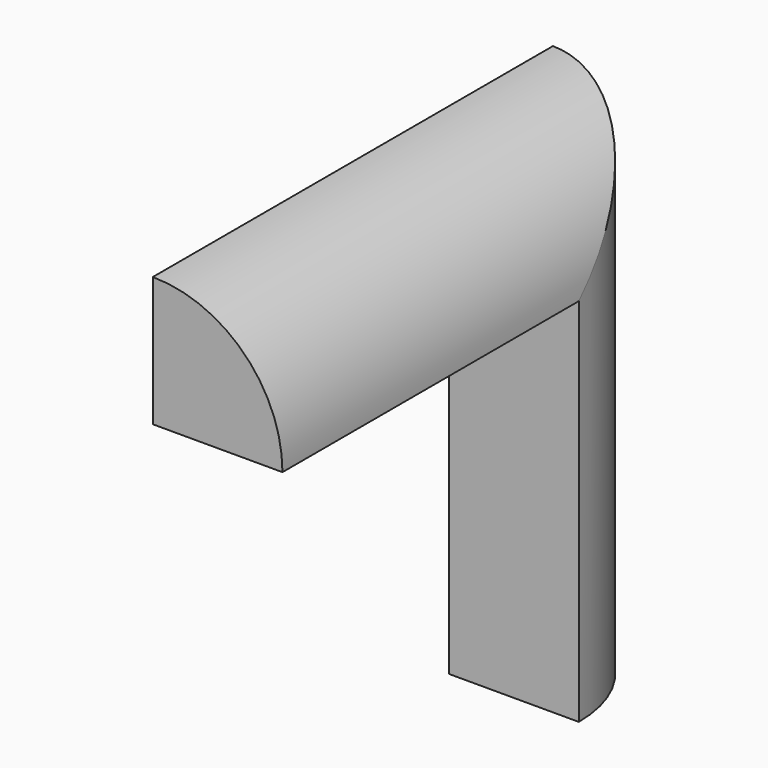
from build123d import *

# Parameters (mm, degrees)
F1_DEPTH      = 15
F3_DEPTH      = 15
F3_DEPTH_BACK = 7
F6_DEPTH      = 20
F7_DEPTH      = 20


with BuildPart() as f1:
    # F0 (on Top) → F1 (new body)
    with BuildSketch(Plane.XY):
        with BuildLine():
            Line((0, 0), (7, 0))
            ThreePointArc((7, 0), (4.9497474683, 4.9497474683), (0, 7))
            Line((0, 7), (0, 0))
        make_face()
    extrude(amount=F1_DEPTH)


with BuildPart() as f3:
    # F2 (on face) → F3 (new body, two sides)
    with BuildSketch(Plane.XZ) as f3_sk:
        with BuildLine():
            ThreePointArc((7, 8), (4.9497474683, 12.9497474683), (0, 15))
            Line((0, 15), (0, 8))
            Line((0, 8), (7, 8))
        make_face()
    extrude(amount=F3_DEPTH)
    extrude(f3_sk.sketch, amount=-F3_DEPTH_BACK)

    # F4: intersect F1
    add(f1.part, mode=Mode.INTERSECT)

    # F6 (add): a face of the model
    f6_faces = [f3.faces().sort_by_distance(p)[0] for p in [
        (2.970892271, 0, 10.970892271),
    ]]
    extrude(f6_faces, amount=F6_DEPTH)

    # F5 (on face) → F7 (join)
    with BuildSketch(Plane(origin=(0, 0, 8), x_dir=(1, 0, 0), z_dir=(0, 0, -1))):
        with BuildLine():
            ThreePointArc((0, -7), (4.9497474683, -4.9497474683), (7, 0))
            Line((7, 0), (0, 0))
            Line((0, 0), (0, -7))
        make_face()
    extrude(amount=F7_DEPTH)


solid = f3.part
